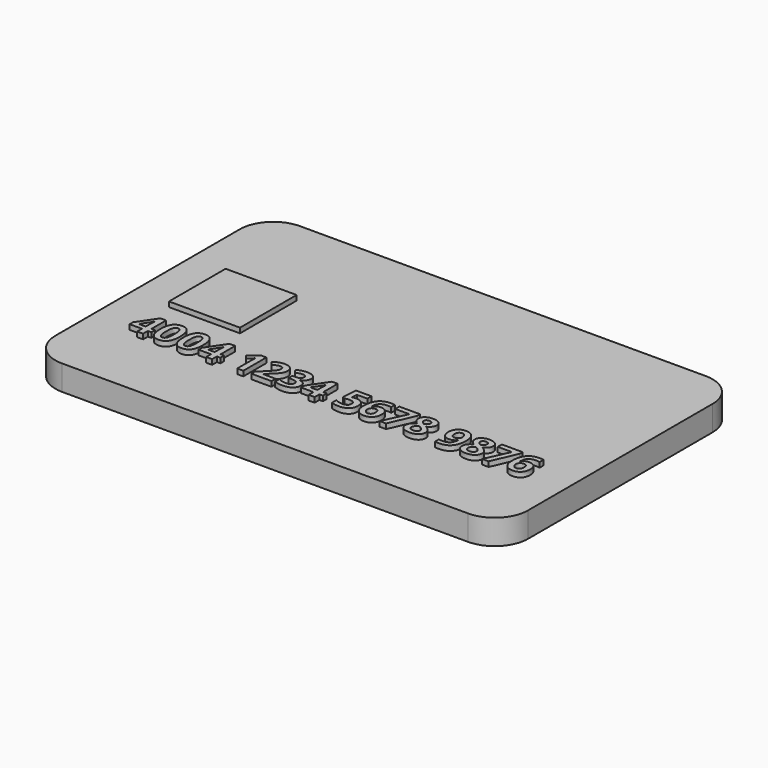
from build123d import *

# Parameters (mm, degrees)
F1_TEXT_SIZE = 2.4132350862
F2_DEPTH     = 1.8
F0_W         = 4.2494963855
F0_H         = 4.2364193359
F0_W_2       = 1.2988597155
F0_H_2       = 1.3752621599
F3_DEPTH     = 1.8
F4_DEPTH     = 1.5


# Not quite as in the source:
# - Text() gives the source's letters only with a copy of the font that has no kerning and outlines rounded to 1/6400 em; it was checked with that copy


with BuildPart() as f2:
    # F1 (on Top) → F2 (new body)
    with BuildSketch(Plane.XY):
        with Locations((-21.2358850986, -4.9199026544)):
            Text('4004 1234 5678 9876', F1_TEXT_SIZE, font='Open Sans', font_style=FontStyle.BOLD, text_align=(TextAlign.LEFT, TextAlign.BOTTOM))
    extrude(amount=F2_DEPTH)



with BuildPart() as f3:
    # F0 (on Top) → F3 (new body)
    with BuildSketch(Plane.XY):
        with Locations((-19.0727682784, 0.503337651)):
            Rectangle(F0_W, F0_H)
        with Locations((-19.049115479, 0.4058468621)):
            Rectangle(F0_W_2, F0_H_2, mode=Mode.SUBTRACT)
        with Locations((-19.049115479, 0.4058468621)):
            Rectangle(F0_W_2, F0_H_2)
    extrude(amount=F3_DEPTH)


with BuildPart() as f2_1:
    add(f2.part)

    add(f3.part)  # F4 merges F3
    # F0 (on Top) → F4 (join)
    with BuildSketch(Plane.XY):
        with BuildLine():
            Line((2.7616547063, 8.6119692668), (-21.5383452937, 8.6119692668))
            ThreePointArc((-21.5383452937, 8.6119692668), (-22.9525588561, 8.0261828292), (-23.5383452937, 6.6119692668))
            Line((-23.5383452937, 6.6119692668), (-23.5383452937, -7.1880307332))
            ThreePointArc((-23.5383452937, -7.1880307332), (-22.9525588561, -8.6022442956), (-21.5383452937, -9.1880307332))
            Line((-21.5383452937, -9.1880307332), (2.7616547063, -9.1880307332))
            ThreePointArc((2.7616547063, -9.1880307332), (4.1758682687, -8.6022442956), (4.7616547063, -7.1880307332))
            Line((4.7616547063, -7.1880307332), (4.7616547063, 6.6119692668))
            ThreePointArc((4.7616547063, 6.6119692668), (4.1758682687, 8.0261828292), (2.7616547063, 8.6119692668))
        make_face()
        with Locations((-19.0727682784, 0.503337651)):
            Rectangle(F0_W, F0_H, mode=Mode.SUBTRACT)
    extrude(amount=F4_DEPTH)


solid = f2_1.part
